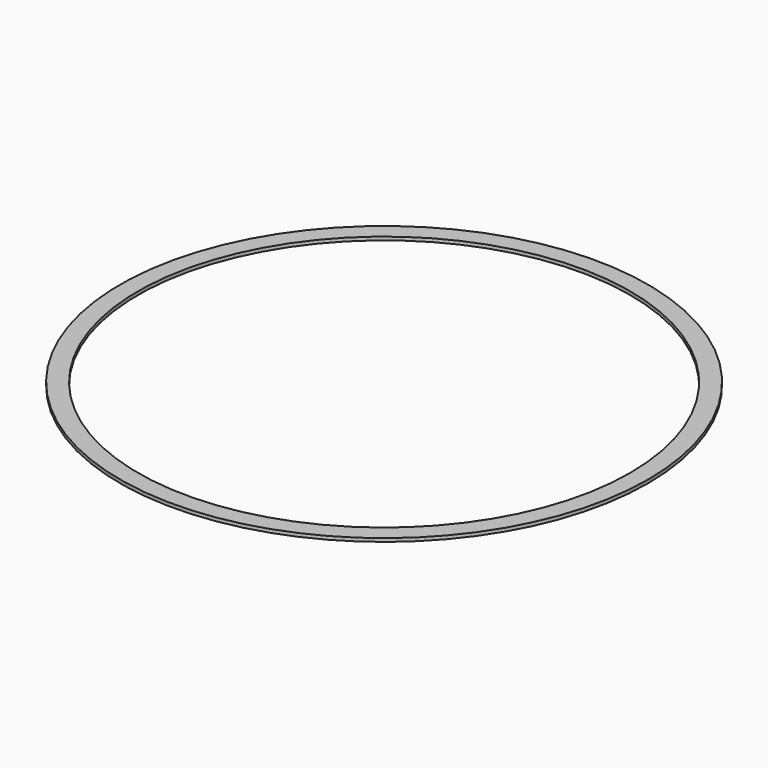
from build123d import *

# Parameters (mm, degrees)
F0_R     = 374.2309
F0_R_2   = 348.8309
F1_DEPTH = 4.7625


# Not quite as in the source:
# - a length typed as a fraction of an inch, garbled in the dataset ("3 / 203.2 mm" for 3/8 in), is restored


with BuildPart() as f1:
    # F0 (on Top) → F1 (new body)
    with BuildSketch(Plane.XY):
        Circle(F0_R)
        Circle(F0_R_2, mode=Mode.SUBTRACT)
    extrude(amount=F1_DEPTH)


solid = f1.part
